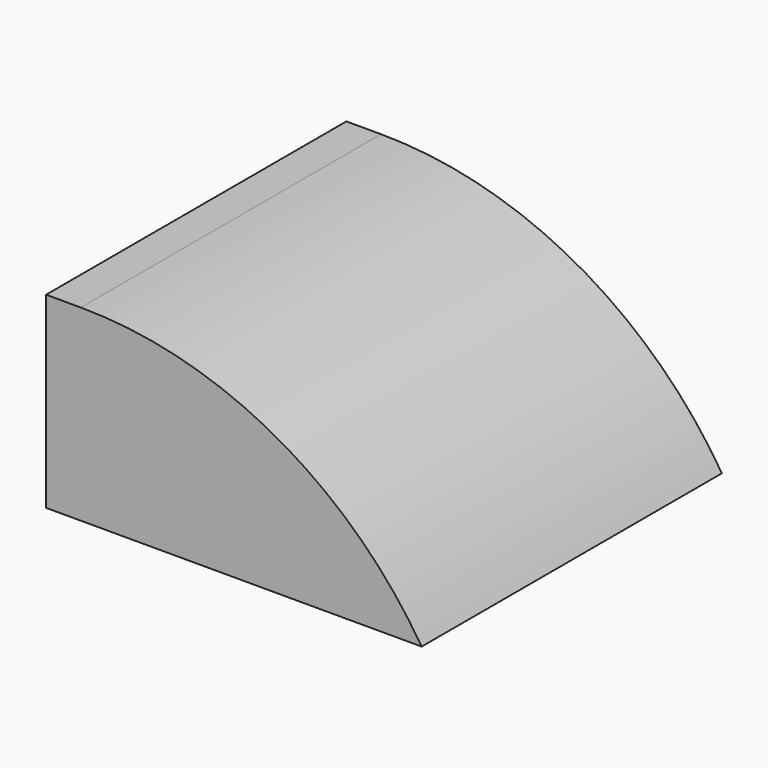
from build123d import *

# Parameters (mm, degrees)
F0_W        = 53.3761642873
F0_H        = 53.3400028944
F1_DEPTH    = 53.34
F4_T1_DEPTH = 591.1352105984


# Not quite as in the source:
# - a fillet or chamfer that OpenCascade refuses, or shapes differently, is made with other operations: its cross-section is extruded or revolved along the edge and cut away or added


with BuildPart() as f1:
    # F0 (on Front) → F1 (new body)
    with BuildSketch(Plane.XZ):
        with Locations((-26.6880821437, 26.6700014472)):
            Rectangle(F0_W, F0_H)
    extrude(amount=F1_DEPTH)

    # F2: F1 across plane


with BuildPart() as f1_1:
    add(f1.part)
    add(f1.part.mirror(Plane.YZ))

    # F3: F1 across face


with BuildPart() as f1_2:
    add(f1_1.part)
    add(f1_1.part.mirror(Plane(origin=(0, -53.34, 26.6700014472), x_dir=(1, 0, 0), z_dir=(0, -1, 0))))

    # F4: fillet of radius 114.6703157856 on 1 edges, made by hand

    # F4_s2 → F4_t1 (cut)
    with BuildSketch(Plane.XZ.offset(-242.2276052992)):
        with BuildLine():
            ThreePointArc((-43.5148778323, 53.3400028944), (11.7866365045, 39.1237753005), (53.3761642873, 0))
            Line((53.3761642873, 0), (53.3761642873, 53.3400028944))
            Line((53.3761642873, 53.3400028944), (-43.5148778323, 53.3400028944))
        make_face()
    extrude(amount=F4_T1_DEPTH, mode=Mode.SUBTRACT)


solid = f1_2.part
